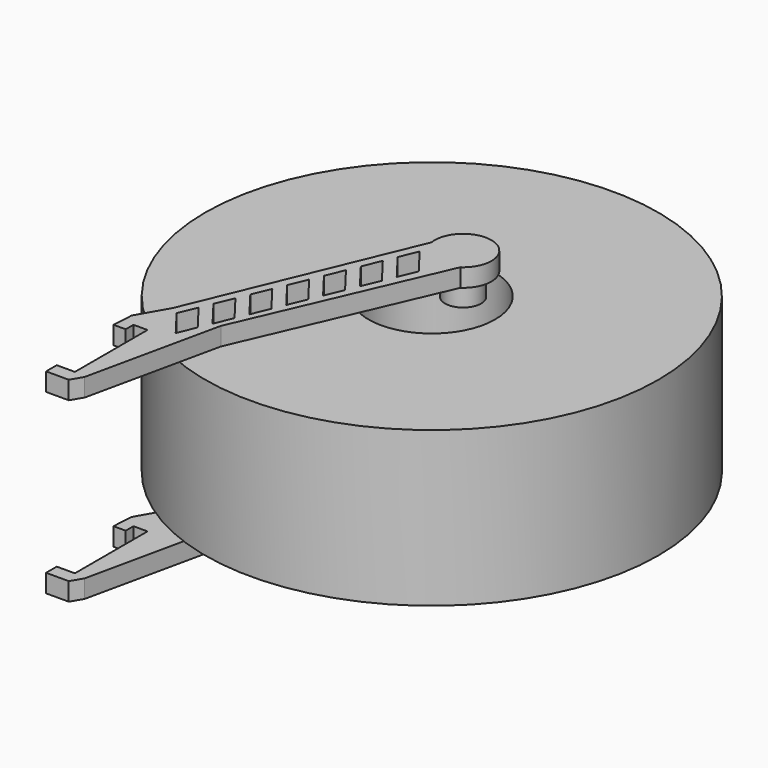
from build123d import *

# Parameters (mm, degrees)
F1_DEPTH  = 8
F2_R      = 8
F3_DEPTH  = 10
F5_DEPTH  = 8.001
F9_R      = 100.076
F9_R_2    = 27.94
F10_DEPTH = 68.326


# Not quite as in the source:
# - ends of sketch curves that miss each other by under 0.0002 mm in the source are joined


with BuildPart() as f1:
    # F0 (on Top) → F1 (new body)
    with BuildSketch(Plane.XY):
        with BuildLine():
            Line((-56.2, -77), (-50, -77))
            Line((-50, -77), (-50, -117.1))
            Line((-50, -117.1), (-56.2, -117.1))
            Line((-56.2, -117.1), (-58, -117.1))
            Line((-58, -117.1), (-58, -123))
            Line((-58, -123), (-48, -123))
            Line((-48, -123), (-45, -118))
            Line((-45, -118), (-32.151355, -58.86091))
            Line((-32.151355, -58.86091), (5, 27))
            ThreePointArc((5, 27), (2.8675773473, 48.8107332803), (-14.3893886651, 35.3032370547))
            Line((-14.3893886651, 35.3032370547), (-53.48139, -58.88472))
            Line((-53.48139, -58.88472), (-61, -72))
            Line((-61, -72), (-61.6, -81.3))
            Line((-61.6, -81.3), (-56.2, -81.3))
            Line((-56.2, -81.3), (-56.2, -77))
        make_face()
    extrude(amount=F1_DEPTH)

    # F2 (on face) → F3 (join)
    with BuildSketch(Plane.XY.offset(8)):
        with Locations((-2.053159, 37.320026)):
            Circle(F2_R)
    extrude(amount=F3_DEPTH)

    # F4 (on face) → F5 (cut, through all)
    with BuildSketch(Plane.XY.offset(8)):
        Polygon((-13.327761602, 27.4264252315), (-16.6475556231, 19.4277398609), (-7.6019353238, 7.6219778501), (-4.2821413027, 15.6206632207), align=None)
        Polygon((-22.2059391411, 6.0354147205), (-13.1603188418, -5.7703472903), (-9.8405248207, 2.2283380803), (-18.88614512, 14.0341000911), align=None)
        Polygon((-27.7643226591, -7.3569104199), (-18.7187023598, -19.1626724307), (-15.3989083387, -11.1639870601), (-24.444528638, 0.6417749506), align=None)
        Polygon((-33.3227061771, -20.7492355604), (-24.2770858777, -32.5549975712), (-20.9572918567, -24.5563122006), (-30.002912156, -12.7505501898), align=None)
        Polygon((-38.8810896951, -34.1415607008), (-29.8354693957, -45.9473227116), (-26.5156753747, -37.948637341), (-35.561295674, -26.1428753302), align=None)
        Polygon((-44.439473213, -47.5338858412), (-35.3938529137, -59.339647852), (-32.0740588927, -51.3409624814), (-41.119679192, -39.5352004706), align=None)
        Polygon((-49.997856731, -60.9262109817), (-40.9522364317, -72.7319729924), (-37.6324424106, -64.7332876219), (-46.67806271, -52.9275256111), align=None)
    extrude(amount=-F5_DEPTH, mode=Mode.SUBTRACT)


with BuildPart() as f6_1:
    # F6: instance of F1
    add(f1.part.mirror(Plane.XY))


with BuildPart() as f10:
    # F9 (on offset) → F10 (new body)
    with BuildSketch(Plane.XY.offset(9)):
        with Locations((0, 17.4860113252)):
            Circle(F9_R)
        with Locations((0, 17.4860113252)):
            Circle(F9_R_2, mode=Mode.SUBTRACT)
    extrude(amount=F10_DEPTH)


with BuildPart() as f6_1_1:
    # F11: moved
    add(f6_1.part.moved(Location((0, 0, 86.326))))


solid = Compound([f1.part, f10.part, f6_1_1.part])
